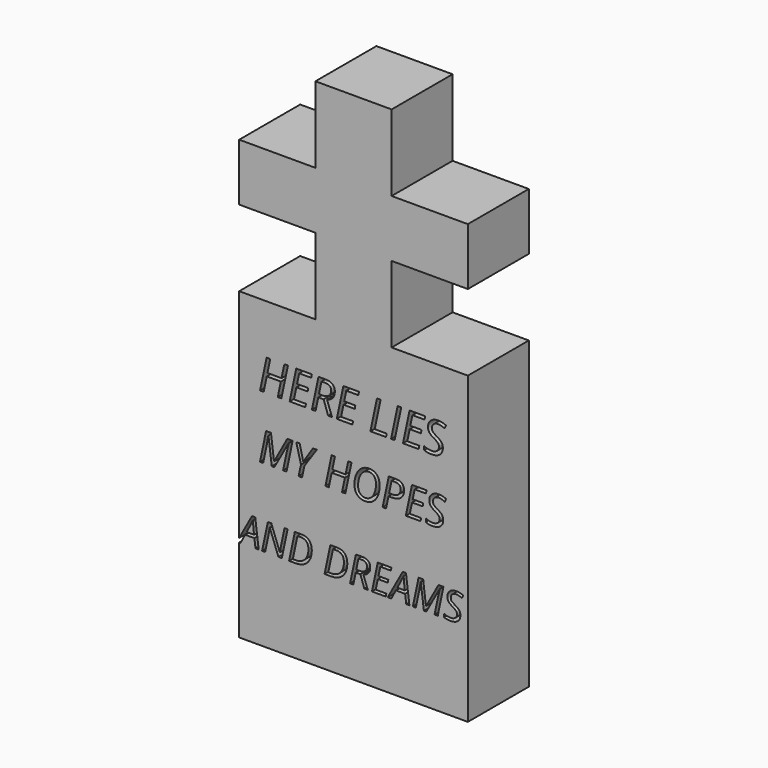
from build123d import *

# Parameters (mm, degrees)
F1_DEPTH       = 25.4
F2_TEXT_SIZE   = 14.5319316313
F2_TEXT_SIZE_2 = 13.6348386231
F2_TEXT_SIZE_3 = 12.7838943064
F3_DEPTH       = 12.7


# Not quite as in the source:
# - Text() gives the source's letters only with a copy of the font that has no kerning and outlines rounded to 1/6400 em; it was checked with that copy


with BuildPart() as f1:
    # F0 (on Front) → F1 (new body)
    with BuildSketch(Plane.XZ):
        Polygon((-12.7, 73.7199598691), (-38.1, 73.7199598691), (-38.1, -27.8800401309), (38.1, -27.8800401309), (38.1, 73.7199598691), (12.7, 73.7199598691), (12.7, 99.1199598691), (38.1, 99.1199598691), (38.1, 118.1699598691), (12.7, 118.1699598691), (12.7, 143.5699598691), (-12.7, 143.5699598691), (-12.7, 118.1699598691), (-38.1, 118.1699598691), (-38.1, 99.1199598691), (-12.7, 99.1199598691), align=None)
    extrude(amount=F1_DEPTH)

    # F2 (on face) → F3 (cut)
    with BuildSketch(Plane.XZ.offset(25.4)):
        with Locations((-31.75, 46.830737517)):
            Text('HERE LIES', F2_TEXT_SIZE, font='Open Sans', font_style=FontStyle.ITALIC, text_align=(TextAlign.LEFT, TextAlign.BOTTOM))
        with Locations((-31.75, 25.8855789108)):
            Text('MY HOPES', F2_TEXT_SIZE_2, font='Open Sans', font_style=FontStyle.ITALIC, text_align=(TextAlign.LEFT, TextAlign.BOTTOM))
        with Locations((-38.1, 0)):
            Text('AND DREAMS', F2_TEXT_SIZE_3, font='Open Sans', font_style=FontStyle.ITALIC, text_align=(TextAlign.LEFT, TextAlign.BOTTOM))
    extrude(amount=-F3_DEPTH, mode=Mode.SUBTRACT)


solid = f1.part
